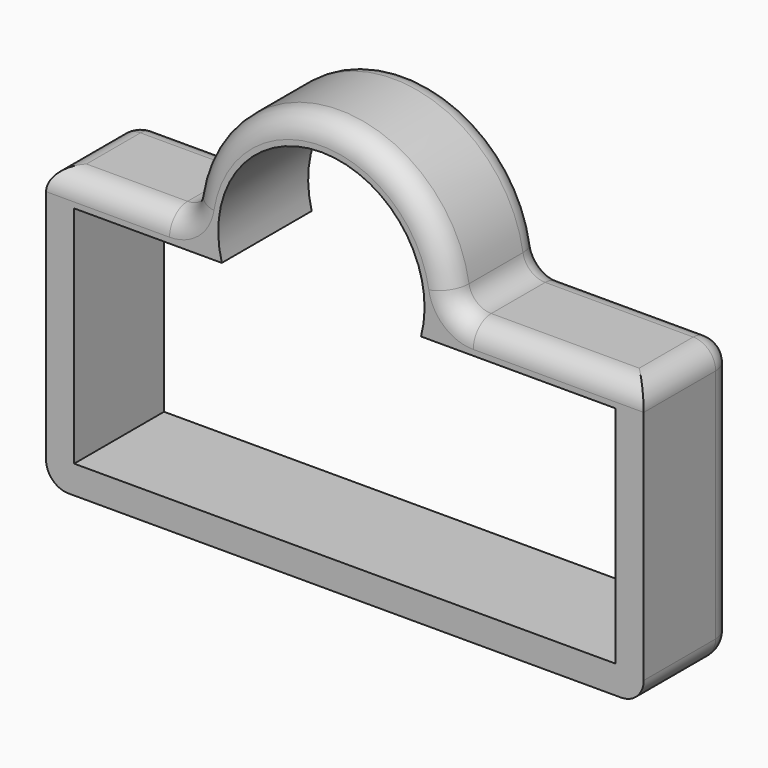
from build123d import *

# Parameters (mm, degrees)
F1_DEPTH = 25.4
F2_R     = 5.08


with BuildPart() as f1:
    # F0 (on Front) → F1 (new body)
    with BuildSketch(Plane.XZ):
        with BuildLine():
            Line((72.8656170726, 0.2934658736), (29.6668574194, 0.2934658736))
            ThreePointArc((29.6668574194, 0.2934658736), (0, 29.6683088726), (-29.6668574194, 0.2934658736))
            Line((-29.6668574194, 0.2934658736), (-62.2401205659, 0.2934658736))
            Line((-62.2401205659, 0.2934658736), (-62.2401205659, -63.2065341264))
            Line((-62.2401205659, -63.2065341264), (72.8656170726, -63.2065341264))
            Line((72.8656170726, -63.2065341264), (72.8656170726, 0.2934658736))
        make_face()
        with BuildLine():
            ThreePointArc((-22.5180355061, -6.0565341264), (0, 23.3183088726), (22.5180355061, -6.0565341264))
            Line((22.5180355061, -6.0565341264), (66.5156170726, -6.0565341264))
            Line((66.5156170726, -6.0565341264), (66.5156170726, -56.8565341264))
            Line((66.5156170726, -56.8565341264), (-55.8901205659, -56.8565341264))
            Line((-55.8901205659, -56.8565341264), (-55.8901205659, -6.0565341264))
            Line((-55.8901205659, -6.0565341264), (-22.5180355061, -6.0565341264))
        make_face(mode=Mode.SUBTRACT)
    extrude(amount=F1_DEPTH)

    # F2
    f2_edges = [f1.edges().sort_by_distance(p)[0] for p in [
        (51.266237, 0, 0.293466),
        (0, 0, 29.668309),
        (-45.953489, 0, 0.293466),
        (-62.240121, 0, -31.456534),
        (5.312748, 0, -63.206534),
        (72.865617, 0, -31.456534),
        (72.865617, -12.7, 0.293466),
        (-62.240121, -12.7, 0.293466),
        (29.666857, -12.7, 0.293466),
        (-29.666857, -12.7, 0.293466),
        (-45.953489, -25.4, 0.293466),
        (-62.240121, -12.7, -63.206534),
        (72.865617, -12.7, -63.206534),
        (51.266237, -25.4, 0.293466),
        (0, -25.4, 29.668309),
    ]]
    fillet(f2_edges, radius=F2_R)


solid = f1.part
